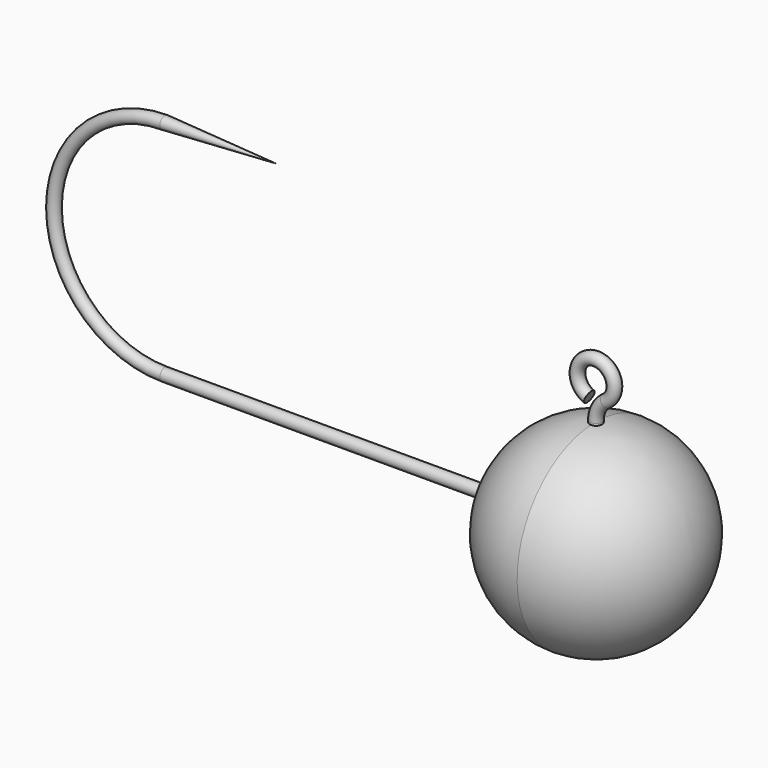
from build123d import *

# Parameters (mm, degrees)
F3_R     = 0.25
F5_SIZE2 = 0.24999
F5_SIZE  = 4.49999


# Not quite as in the source:
# - a fillet or chamfer is up to 0.001 mm smaller than in the source, because OpenCascade refuses the exact size


with BuildPart() as f1:
    # F0 (on Front) → F1 (revolve)
    with BuildSketch(Plane.XZ):
        with BuildLine():
            Line((-1, 0), (4, 0))
            ThreePointArc((4, 0), (2.8284271247, 2.8284271247), (0, 4))
            Line((0, 4), (0, 1))
            ThreePointArc((0, 1), (-0.2928932188, 0.2928932188), (-1, 0))
        make_face()
        with BuildLine():
            Line((0, 1), (0, 4))
            ThreePointArc((0, 4), (-2.8284271247, 2.8284271247), (-4, 0))
            Line((-4, 0), (-1, 0))
            ThreePointArc((-1, 0), (-0.2928932188, 0.2928932188), (0, 1))
        make_face()
    revolve(axis=Axis((-9.25, 0, 0), (-1, 0, 0)))


with BuildPart() as f4:
    # F4: sweep along a path in F0
    with BuildLine(Plane.XZ) as f4_path:
        Line((-13, 9), (-17.5, 9))
        ThreePointArc((-17.5, 9), (-22, 4.5), (-17.5, 0))
        Line((-17.5, 0), (-1, 0))
        ThreePointArc((-1, 0), (-0.2928932188, 0.2928932188), (0, 1))
        Line((0, 1), (0, 4.0638593384))
        ThreePointArc((0, 4.0638593384), (0.1135947396, 4.5267693883), (0.4285714286, 4.884511145))
        ThreePointArc((0.4285714286, 4.884511145), (-0.0889535051, 6.2447061662), (-0.2715447628, 4.8008838138))
    # F3 (on plane+point) → F4 (sweep)
    with BuildSketch(Plane.YZ.offset(-17.5)):
        Circle(F3_R)
    sweep(path=f4_path.line)

    # F5 (size 4.5 and 0.25 in the source; OpenCascade refuses exactly that, so slightly less here)
    f5_edges = [f4.edges().sort_by_distance(p)[0] for p in [
        (-13, -0.25, 9),
    ]]
    chamfer(f5_edges, length=F5_SIZE, length2=F5_SIZE2)


solid = Compound([f1.part, f4.part])
